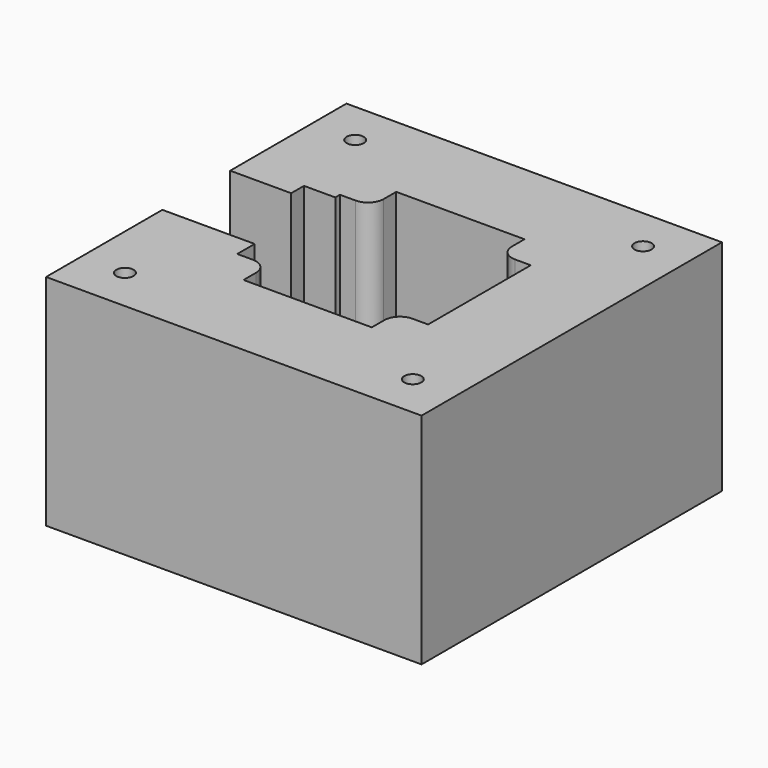
from build123d import *

# Parameters (mm, degrees)
F0_R     = 2.75
F0_W     = 10
F0_H     = 5.1
F1_DEPTH = 70
F2_DEPTH = 45


# Not quite as in the source:
# - a feature names something its author has since deleted; it is built from what else it names


with BuildPart() as f1:
    # F0 (on Top) → F1 (new body)
    with BuildSketch(Plane.XY):
        with BuildLine():
            Line((-60, -60), (60, -60))
            Line((60, -60), (60, 60))
            Line((60, 60), (-60, 60))
            Line((-60, 60), (-60, 13.55))
            Line((-60, 13.55), (-40.5, 13.55))
            Line((-40.5, 13.55), (-40.5, 18.65))
            Line((-40.5, 18.65), (-30.5, 18.65))
            Line((-30.5, 18.65), (-30.5, 20.5))
            Line((-30.5, 20.5), (-25.5, 20.5))
            ThreePointArc((-25.5, 20.5), (-21.9644660941, 21.9644660941), (-20.5, 25.5))
            Line((-20.5, 25.5), (-20.5, 30.5))
            Line((-20.5, 30.5), (20.5, 30.5))
            Line((20.5, 30.5), (20.5, 25.5))
            ThreePointArc((20.5, 25.5), (21.9644660941, 21.9644660941), (25.5, 20.5))
            Line((25.5, 20.5), (30.5, 20.5))
            Line((30.5, 20.5), (30.5, -20.5))
            Line((30.5, -20.5), (25.5, -20.5))
            ThreePointArc((25.5, -20.5), (21.9644660941, -21.9644660941), (20.5, -25.5))
            Line((20.5, -25.5), (20.5, -30.5))
            Line((20.5, -30.5), (-20.5, -30.5))
            Line((-20.5, -30.5), (-20.5, -25.5))
            ThreePointArc((-20.5, -25.5), (-21.9644660941, -21.9644660941), (-25.5, -20.5))
            Line((-25.5, -20.5), (-30.5, -20.5))
            Line((-30.5, -20.5), (-30.5, -18.65))
            Line((-30.5, -18.65), (-30.5, -13.55))
            Line((-30.5, -13.55), (-40.5, -13.55))
            Line((-40.5, -13.55), (-60, -13.55))
            Line((-60, -13.55), (-60, -18.65))
            Line((-60, -18.65), (-60, -60))
        make_face()
        with Locations((-46, -46)):
            Circle(F0_R, mode=Mode.SUBTRACT)
        with Locations((46, -46)):
            Circle(F0_R, mode=Mode.SUBTRACT)
        with Locations((-46, 46)):
            Circle(F0_R, mode=Mode.SUBTRACT)
        with Locations((46, 46)):
            Circle(F0_R, mode=Mode.SUBTRACT)
        Polygon((-60, 13.55), (-60, -13.55), (-40.5, -13.55), (-30.5, -13.55), (-30.5, 13.55), (-40.5, 13.55), align=None)
        with BuildLine():
            Line((-30.5, 13.55), (-30.5, -13.55))
            Line((-30.5, -13.55), (-30.5, -18.65))
            Line((-30.5, -18.65), (-30.5, -20.5))
            Line((-30.5, -20.5), (-25.5, -20.5))
            ThreePointArc((-25.5, -20.5), (-21.9644660941, -21.9644660941), (-20.5, -25.5))
            Line((-20.5, -25.5), (-20.5, -30.5))
            Line((-20.5, -30.5), (20.5, -30.5))
            Line((20.5, -30.5), (20.5, -25.5))
            ThreePointArc((20.5, -25.5), (21.9644660941, -21.9644660941), (25.5, -20.5))
            Line((25.5, -20.5), (30.5, -20.5))
            Line((30.5, -20.5), (30.5, 20.5))
            Line((30.5, 20.5), (25.5, 20.5))
            ThreePointArc((25.5, 20.5), (21.9644660941, 21.9644660941), (20.5, 25.5))
            Line((20.5, 25.5), (20.5, 30.5))
            Line((20.5, 30.5), (-20.5, 30.5))
            Line((-20.5, 30.5), (-20.5, 25.5))
            ThreePointArc((-20.5, 25.5), (-21.9644660941, 21.9644660941), (-25.5, 20.5))
            Line((-25.5, 20.5), (-30.5, 20.5))
            Line((-30.5, 20.5), (-30.5, 18.65))
            Line((-30.5, 18.65), (-30.5, 13.55))
        make_face()
        with Locations((-35.5, 16.1)):
            Rectangle(F0_W, F0_H)
    extrude(amount=-F1_DEPTH)

    # F0 (on Top) → F2 (cut)
    with BuildSketch(Plane.XY):
        Polygon((-60, 13.55), (-60, -13.55), (-40.5, -13.55), (-30.5, -13.55), (-30.5, 13.55), (-40.5, 13.55), align=None)
        with BuildLine():
            Line((-30.5, 13.55), (-30.5, -13.55))
            Line((-30.5, -13.55), (-30.5, -18.65))
            Line((-30.5, -18.65), (-30.5, -20.5))
            Line((-30.5, -20.5), (-25.5, -20.5))
            ThreePointArc((-25.5, -20.5), (-21.9644660941, -21.9644660941), (-20.5, -25.5))
            Line((-20.5, -25.5), (-20.5, -30.5))
            Line((-20.5, -30.5), (20.5, -30.5))
            Line((20.5, -30.5), (20.5, -25.5))
            ThreePointArc((20.5, -25.5), (21.9644660941, -21.9644660941), (25.5, -20.5))
            Line((25.5, -20.5), (30.5, -20.5))
            Line((30.5, -20.5), (30.5, 20.5))
            Line((30.5, 20.5), (25.5, 20.5))
            ThreePointArc((25.5, 20.5), (21.9644660941, 21.9644660941), (20.5, 25.5))
            Line((20.5, 25.5), (20.5, 30.5))
            Line((20.5, 30.5), (-20.5, 30.5))
            Line((-20.5, 30.5), (-20.5, 25.5))
            ThreePointArc((-20.5, 25.5), (-21.9644660941, 21.9644660941), (-25.5, 20.5))
            Line((-25.5, 20.5), (-30.5, 20.5))
            Line((-30.5, 20.5), (-30.5, 18.65))
            Line((-30.5, 18.65), (-30.5, 13.55))
        make_face()
        with Locations((-35.5, 16.1)):
            Rectangle(F0_W, F0_H)
    extrude(amount=-F2_DEPTH, mode=Mode.SUBTRACT)


solid = f1.part
